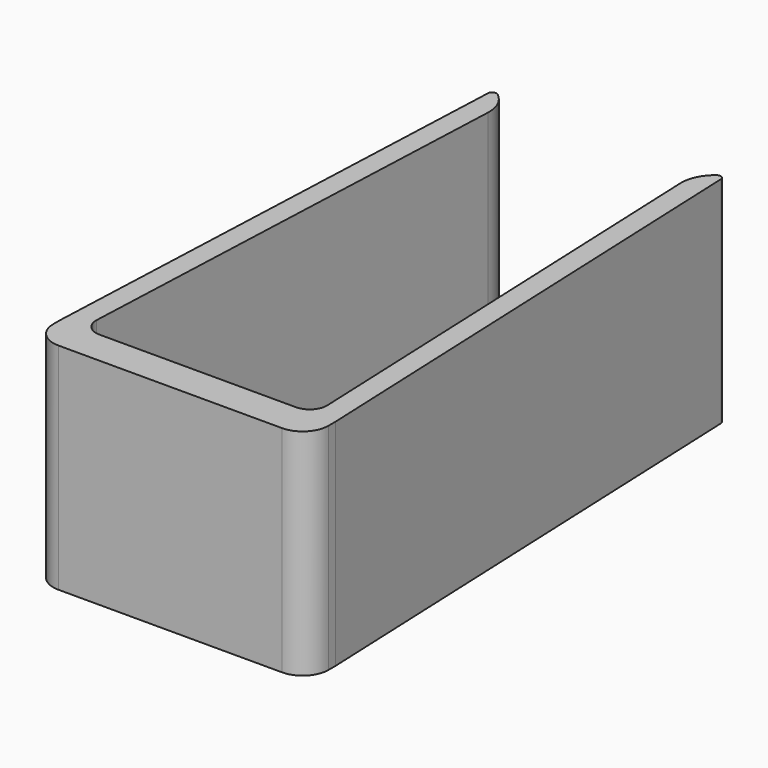
from build123d import *

# Parameters (mm, degrees)
F1_DEPTH    = 25
F2_T1_DEPTH = 44.0569346235
F3_R        = 0.5
F4_R        = 3
F5_R        = 2


# Not quite as in the source:
# - a fillet or chamfer that OpenCascade refuses, or shapes differently, is made with other operations: its cross-section is extruded or revolved along the edge and cut away or added


with BuildPart() as f1:
    # F0 (on Top) → F1 (new body)
    with BuildSketch(Plane.XY):
        Polygon((-13.5, 61.9478940414), (-16, 2), (-13.5, 2), (-11, 61.9478940414), align=None)
        Polygon((13.5, 2), (16, 2), (13.5, 61.9478940414), (11, 61.9478940414), align=None)
        Polygon((-16, -2), (16, -2), (16, 2), (13.5, 2), (-13.5, 2), (-16, 2), align=None)
    extrude(amount=F1_DEPTH)

    # F2: fillet of radius 4 on 2 edges, made by hand

    # F2_s2 → F2_t1 (cut)
    with BuildSketch(Plane.XY.offset(-9.5284673118)):
        with BuildLine():
            ThreePointArc((13.5, 61.9478940414), (11.7478065256, 60.4014195424), (11.1588077885, 58.1398170495))
            Line((11.1588077885, 58.1398170495), (11, 61.9478940414))
            Line((11, 61.9478940414), (13.5, 61.9478940414))
        make_face()
        with BuildLine():
            ThreePointArc((-13.5, 61.9478940414), (-11.7478065256, 60.4014195424), (-11.1588077885, 58.1398170495))
            Line((-11.1588077885, 58.1398170495), (-11, 61.9478940414))
            Line((-11, 61.9478940414), (-13.5, 61.9478940414))
        make_face()
    extrude(amount=F2_T1_DEPTH, mode=Mode.SUBTRACT)

    # F3
    f3_edges = [f1.edges().sort_by_distance(p)[0] for p in [
        (-13.5, 61.947894, 12.5),
        (13.5, 61.947894, 12.5),
    ]]
    fillet(f3_edges, radius=F3_R)

    # F4
    f4_edges = [f1.edges().sort_by_distance(p)[0] for p in [
        (16, -2, 12.5),
        (-16, -2, 12.5),
    ]]
    fillet(f4_edges, radius=F4_R)

    # F5
    f5_edges = [f1.edges().sort_by_distance(p)[0] for p in [
        (-13.5, 2, 12.5),
        (13.5, 2, 12.5),
    ]]
    fillet(f5_edges, radius=F5_R)


solid = f1.part
